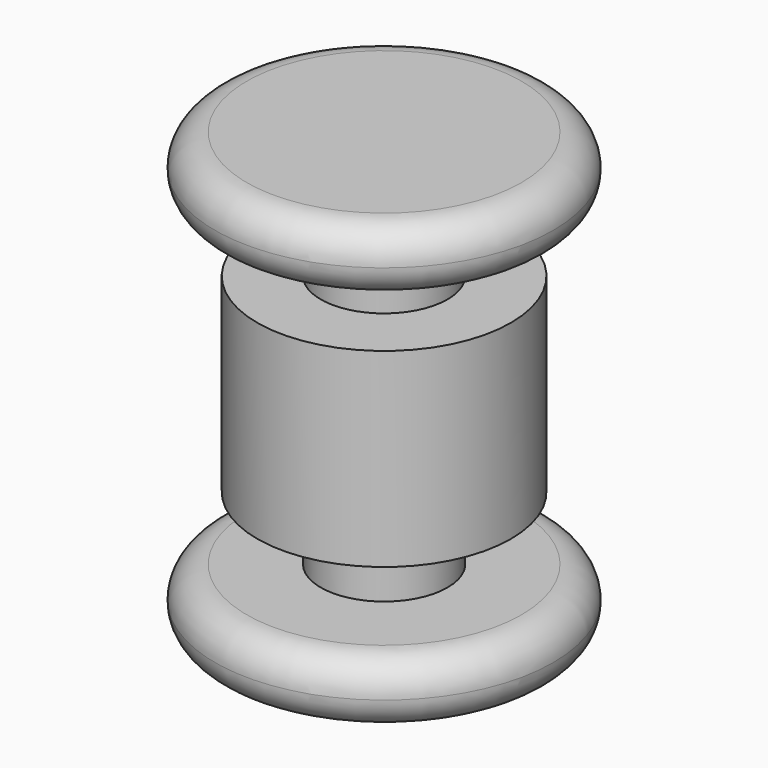
from build123d import *

# Parameters (mm, degrees)
F0_R     = 8
F1_DEPTH = 3
F2_R     = 6
F3_DEPTH = 15
F4_R     = 8
F4_R_2   = 6
F5_DEPTH = 3
F6_R     = 1.49999
F7_W     = 3
F7_H     = 3


# Not quite as in the source:
# - a fillet or chamfer is up to 0.001 mm smaller than in the source, because OpenCascade refuses the exact size


with BuildPart() as f1:
    # F0 (on Top) → F1 (new body)
    with BuildSketch(Plane.XY):
        Circle(F0_R)
    extrude(amount=F1_DEPTH)

    # F2 (on face) → F3 (join)
    with BuildSketch(Plane.XY.offset(3)):
        Circle(F2_R)
    extrude(amount=F3_DEPTH)

    # F4 (on face) → F5 (join)
    with BuildSketch(Plane.XY.offset(18)):
        Circle(F4_R)
        Circle(F4_R_2, mode=Mode.SUBTRACT)
        Circle(F4_R_2)
    extrude(amount=F5_DEPTH)

    # F6 (radius 1.5 in the source; OpenCascade refuses exactly that, so slightly less here)
    f6_edges = [f1.edges().sort_by_distance(p)[0] for p in [
        (-8, 0, 21),
        (-8, 0, 18),
        (-8, 0, 3),
        (-8, 0, 0),
    ]]
    fillet(f6_edges, radius=F6_R)

    # F7 (on Front) → F8 (revolve, cut)
    with BuildSketch(Plane.XZ):
        with Locations((4.5, 4.5)):
            Rectangle(F7_W, F7_H)
        with Locations((4.5, 16.5)):
            Rectangle(F7_W, F7_H)
    revolve(axis=Axis((0, 0, 11.7473863065), (0, 0, 1)), mode=Mode.SUBTRACT)


solid = f1.part
